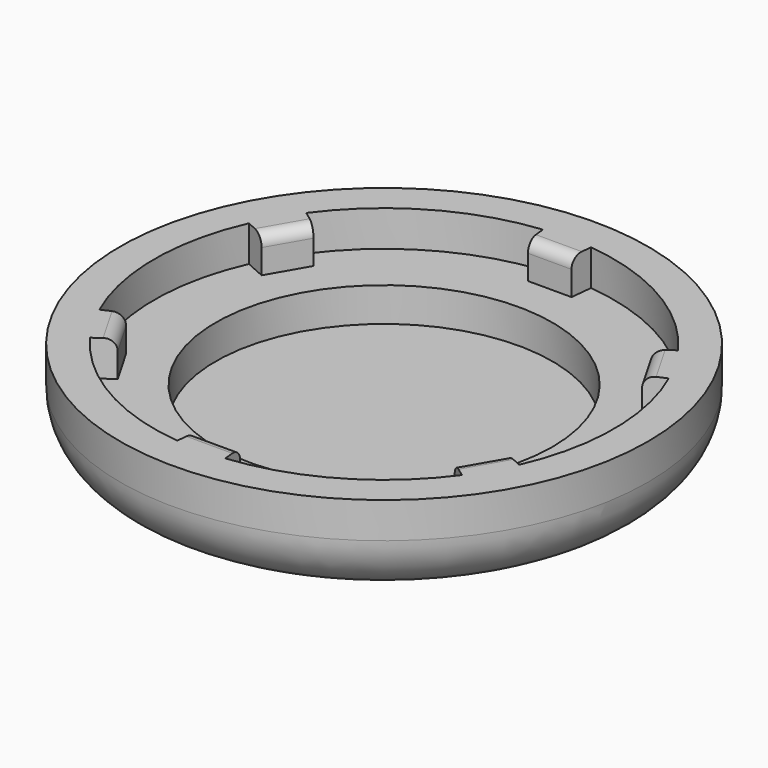
from build123d import *

# Parameters (mm, degrees)
F0_R     = 14.732
F1_DEPTH = 3.175
F2_DEPTH = 2
F3_R     = 9.398
F4_DEPTH = 1.905
F6_R     = 0.635


# Not quite as in the source:
# - a fillet or chamfer that OpenCascade refuses, or shapes differently, is made with other operations: its cross-section is extruded or revolved along the edge and cut away or added


with BuildPart() as f1:
    # F0 (on Top) → F1 (new body)
    with BuildSketch(Plane.XY):
        Circle(F0_R)
        with BuildLine():
            ThreePointArc((-10.3772609868, 7.5395214312), (-6.4135, 11.1085078543), (-1.3407865983, 12.7567323519))
            Line((-1.3407865983, 12.7567323519), (-1.214689647, 11.557))
            Line((-1.214689647, 11.557), (1.214689647, 11.557))
            Line((1.214689647, 11.557), (1.3407865983, 12.7567323519))
            ThreePointArc((1.3407865983, 12.7567323519), (6.4135, 11.1085078543), (10.3772609868, 7.5395214312))
            Line((10.3772609868, 7.5395214312), (9.4013107681, 6.830452092))
            Line((9.4013107681, 6.830452092), (10.616000415, 4.726547908))
            Line((10.616000415, 4.726547908), (11.7180475852, 5.2172109207))
            ThreePointArc((11.7180475852, 5.2172109207), (12.827, 0), (11.7180475852, -5.2172109207))
            Line((11.7180475852, -5.2172109207), (10.616000415, -4.726547908))
            Line((10.616000415, -4.726547908), (9.4013107681, -6.830452092))
            Line((9.4013107681, -6.830452092), (10.3772609868, -7.5395214312))
            ThreePointArc((10.3772609868, -7.5395214312), (6.4135, -11.1085078543), (1.3407865983, -12.7567323519))
            Line((1.3407865983, -12.7567323519), (1.214689647, -11.557))
            Line((1.214689647, -11.557), (-1.214689647, -11.557))
            Line((-1.214689647, -11.557), (-1.3407865983, -12.7567323519))
            ThreePointArc((-1.3407865983, -12.7567323519), (-6.4135, -11.1085078543), (-10.3772609868, -7.5395214312))
            Line((-10.3772609868, -7.5395214312), (-9.4013107681, -6.830452092))
            Line((-9.4013107681, -6.830452092), (-10.616000415, -4.726547908))
            Line((-10.616000415, -4.726547908), (-11.7180475852, -5.2172109207))
            ThreePointArc((-11.7180475852, -5.2172109207), (-12.827, 0), (-11.7180475852, 5.2172109207))
            Line((-11.7180475852, 5.2172109207), (-10.616000415, 4.726547908))
            Line((-10.616000415, 4.726547908), (-9.4013107681, 6.830452092))
            Line((-9.4013107681, 6.830452092), (-10.3772609868, 7.5395214312))
        make_face(mode=Mode.SUBTRACT)
        with BuildLine():
            Line((-1.214689647, 11.557), (-1.3407865983, 12.7567323519))
            ThreePointArc((-1.3407865983, 12.7567323519), (-6.4135, 11.1085078543), (-10.3772609868, 7.5395214312))
            Line((-10.3772609868, 7.5395214312), (-9.4013107681, 6.830452092))
            Line((-9.4013107681, 6.830452092), (-10.616000415, 4.726547908))
            Line((-10.616000415, 4.726547908), (-11.7180475852, 5.2172109207))
            ThreePointArc((-11.7180475852, 5.2172109207), (-12.827, 0), (-11.7180475852, -5.2172109207))
            Line((-11.7180475852, -5.2172109207), (-10.616000415, -4.726547908))
            Line((-10.616000415, -4.726547908), (-9.4013107681, -6.830452092))
            Line((-9.4013107681, -6.830452092), (-10.3772609868, -7.5395214312))
            ThreePointArc((-10.3772609868, -7.5395214312), (-6.4135, -11.1085078543), (-1.3407865983, -12.7567323519))
            Line((-1.3407865983, -12.7567323519), (-1.214689647, -11.557))
            Line((-1.214689647, -11.557), (1.214689647, -11.557))
            Line((1.214689647, -11.557), (1.3407865983, -12.7567323519))
            ThreePointArc((1.3407865983, -12.7567323519), (6.4135, -11.1085078543), (10.3772609868, -7.5395214312))
            Line((10.3772609868, -7.5395214312), (9.4013107681, -6.830452092))
            Line((9.4013107681, -6.830452092), (10.616000415, -4.726547908))
            Line((10.616000415, -4.726547908), (11.7180475852, -5.2172109207))
            ThreePointArc((11.7180475852, -5.2172109207), (12.827, 0), (11.7180475852, 5.2172109207))
            Line((11.7180475852, 5.2172109207), (10.616000415, 4.726547908))
            Line((10.616000415, 4.726547908), (9.4013107681, 6.830452092))
            Line((9.4013107681, 6.830452092), (10.3772609868, 7.5395214312))
            ThreePointArc((10.3772609868, 7.5395214312), (6.4135, 11.1085078543), (1.3407865983, 12.7567323519))
            Line((1.3407865983, 12.7567323519), (1.214689647, 11.557))
            Line((1.214689647, 11.557), (-1.214689647, 11.557))
        make_face()
    extrude(amount=-F1_DEPTH)

    # F0 (on Top) → F2 (join)
    with BuildSketch(Plane.XY):
        Circle(F0_R)
        with BuildLine():
            ThreePointArc((-10.3772609868, 7.5395214312), (-6.4135, 11.1085078543), (-1.3407865983, 12.7567323519))
            Line((-1.3407865983, 12.7567323519), (-1.214689647, 11.557))
            Line((-1.214689647, 11.557), (1.214689647, 11.557))
            Line((1.214689647, 11.557), (1.3407865983, 12.7567323519))
            ThreePointArc((1.3407865983, 12.7567323519), (6.4135, 11.1085078543), (10.3772609868, 7.5395214312))
            Line((10.3772609868, 7.5395214312), (9.4013107681, 6.830452092))
            Line((9.4013107681, 6.830452092), (10.616000415, 4.726547908))
            Line((10.616000415, 4.726547908), (11.7180475852, 5.2172109207))
            ThreePointArc((11.7180475852, 5.2172109207), (12.827, 0), (11.7180475852, -5.2172109207))
            Line((11.7180475852, -5.2172109207), (10.616000415, -4.726547908))
            Line((10.616000415, -4.726547908), (9.4013107681, -6.830452092))
            Line((9.4013107681, -6.830452092), (10.3772609868, -7.5395214312))
            ThreePointArc((10.3772609868, -7.5395214312), (6.4135, -11.1085078543), (1.3407865983, -12.7567323519))
            Line((1.3407865983, -12.7567323519), (1.214689647, -11.557))
            Line((1.214689647, -11.557), (-1.214689647, -11.557))
            Line((-1.214689647, -11.557), (-1.3407865983, -12.7567323519))
            ThreePointArc((-1.3407865983, -12.7567323519), (-6.4135, -11.1085078543), (-10.3772609868, -7.5395214312))
            Line((-10.3772609868, -7.5395214312), (-9.4013107681, -6.830452092))
            Line((-9.4013107681, -6.830452092), (-10.616000415, -4.726547908))
            Line((-10.616000415, -4.726547908), (-11.7180475852, -5.2172109207))
            ThreePointArc((-11.7180475852, -5.2172109207), (-12.827, 0), (-11.7180475852, 5.2172109207))
            Line((-11.7180475852, 5.2172109207), (-10.616000415, 4.726547908))
            Line((-10.616000415, 4.726547908), (-9.4013107681, 6.830452092))
            Line((-9.4013107681, 6.830452092), (-10.3772609868, 7.5395214312))
        make_face(mode=Mode.SUBTRACT)
    extrude(amount=F2_DEPTH)

    # F3 (on face) → F4 (cut)
    with BuildSketch(Plane.XY):
        Circle(F3_R)
    extrude(amount=-F4_DEPTH, mode=Mode.SUBTRACT)

    # F5: fillet of radius 3.175 on 1 edges, made by hand

    # F5_s1 → F5_t2 (revolve, cut)
    with BuildSketch(Plane.XZ):
        with BuildLine():
            ThreePointArc((14.732, 0), (13.8020640303, -2.2450640303), (11.557, -3.175))
            Line((11.557, -3.175), (14.732, -3.175))
            Line((14.732, -3.175), (14.732, 0))
        make_face()
    revolve(axis=Axis((0, 0, -3.175), (0, 0, 1)), mode=Mode.SUBTRACT)

    # F6
    f6_edges = [f1.edges().sort_by_distance(p)[0] for p in [
        (0, 11.557, 2),
        (10.008656, -5.7785, 2),
        (-10.008656, 5.7785, 2),
        (-10.008656, -5.7785, 2),
        (0, -11.557, 2),
        (10.008656, 5.7785, 2),
    ]]
    fillet(f6_edges, radius=F6_R)


solid = f1.part
